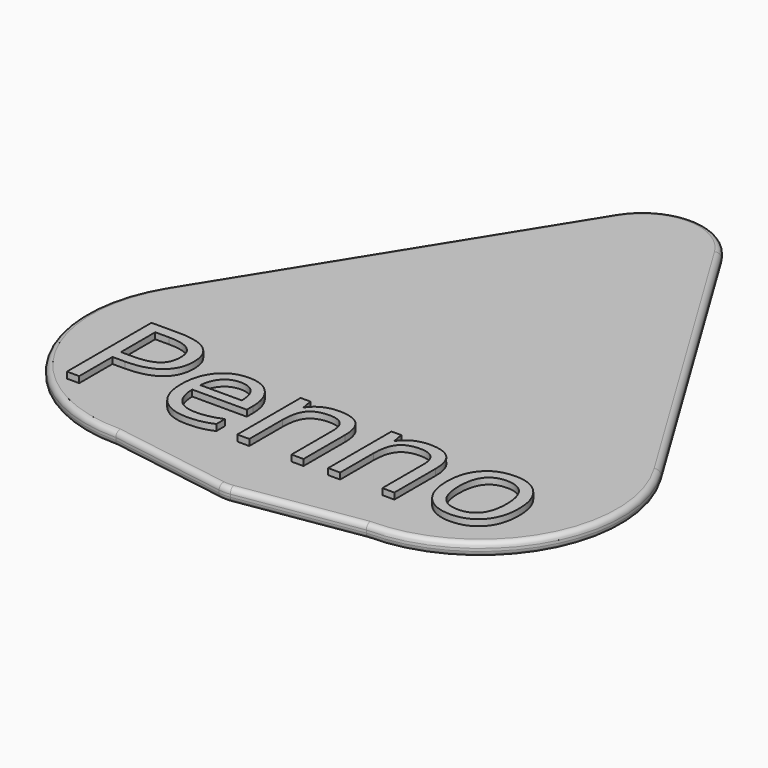
from build123d import *

# Parameters (mm, degrees)
F1_DEPTH     = 0.75
F2_R         = 0.3
F3_TEXT_SIZE = 8.3242287082
F4_DEPTH     = 0.35


# Not quite as in the source:
# - Text() gives the source's letters only with a copy of the font that has no kerning and outlines rounded to 1/6400 em; it was checked with that copy


with BuildPart() as f1:
    # F0 (on Top) → F1 (new body)
    with BuildSketch(Plane.XY):
        with BuildLine():
            ThreePointArc((28.5764611286, -0.0004187508), (35.5507607242, 4.0804159043), (35.4097939417, 12.1596605903))
            Line((35.4097939417, 12.1596605903), (24.5952321598, 29.9234919771))
            ThreePointArc((24.5952321598, 29.9234919771), (21.6225781062, 31.6034164312), (18.6338332418, 29.9522888077))
            Line((18.6338332418, 29.9522888077), (7.6056713814, 12.225464446))
            ThreePointArc((7.6056713814, 12.225464446), (7.4257161114, 4.0776940705), (14.4819868729, 0))
            Line((14.4819868729, 0), (21.1514078331, -1.0717175252))
            ThreePointArc((21.1514078331, -1.0717175252), (21.4658679186, -1.0970476205), (21.7803989603, -1.0726143869))
            Line((21.7803989603, -1.0726143869), (28.5764611286, -0.0004187508))
        make_face()
    extrude(amount=F1_DEPTH)

    # F2
    f2_edges = [f1.edges().sort_by_distance(p)[0] for p in [
        (7.425716, 4.077694, 0.75),
        (17.816697, -0.535859, 0.75),
        (25.17843, -0.536517, 0.75),
        (21.465868, -1.097048, 0.75),
        (35.550761, 4.080416, 0.75),
        (30.002513, 21.041576, 0.75),
        (13.119752, 21.088877, 0.75),
        (21.622578, 31.603416, 0.75),
        (25.17843, -0.536517, 0),
        (35.550761, 4.080416, 0),
        (30.002513, 21.041576, 0),
        (21.622578, 31.603416, 0),
        (13.119752, 21.088877, 0),
        (7.425716, 4.077694, 0),
        (17.816697, -0.535859, 0),
        (21.465868, -1.097048, 0),
    ]]
    fillet(f2_edges, radius=F2_R)

    # F3 (on face) → F4 (join)
    with BuildSketch(Plane.XY.offset(0.75)):
        with Locations((8.8589425069, 2.5744373579)):
            Text('Penno', F3_TEXT_SIZE, font='Open Sans', text_align=(TextAlign.LEFT, TextAlign.BOTTOM))
    extrude(amount=F4_DEPTH)


solid = f1.part
